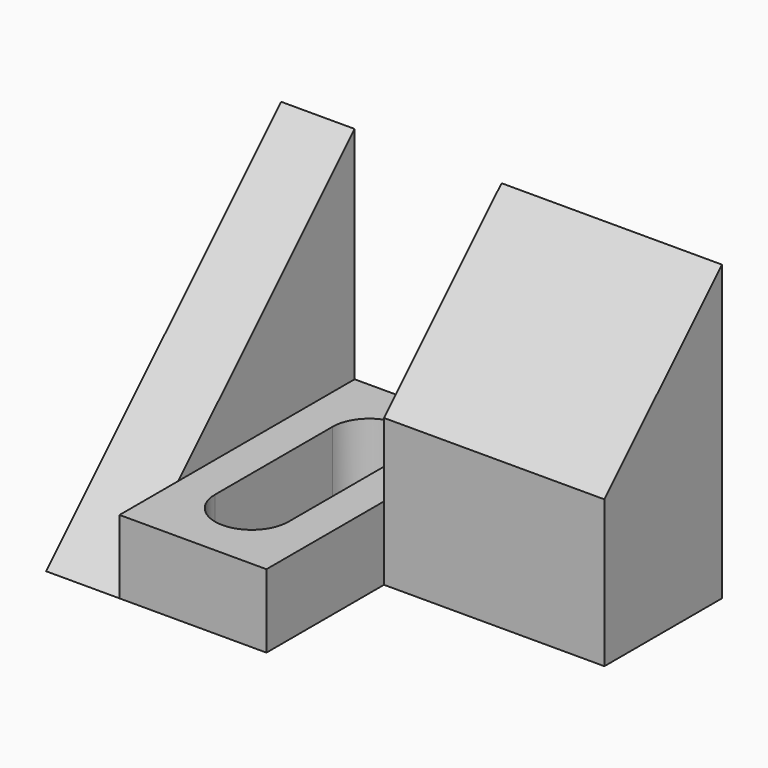
from build123d import *

# Parameters (mm, degrees)
F0_W     = 6.35
F0_H     = 25.4
F1_DEPTH = 25.4
F0_W_2   = 19.05
F0_H_2   = 12.7
F2_DEPTH = 25.4
F3_DEPTH = 6.35
F5_DEPTH = 38.101


# Not quite as in the source:
# - a feature of the source that left no trace in its solid (it failed there, or was rolled back) is left out


with BuildPart() as f1:
    # F0 (on Top) → F1 (new body)
    with BuildSketch(Plane.XY):
        with Locations((3.175, 12.7)):
            Rectangle(F0_W, F0_H)
    extrude(amount=F1_DEPTH)


with BuildPart() as f2:
    # F0 (on Top) → F2 (new body)
    with BuildSketch(Plane.XY):
        with Locations((28.575, 19.05)):
            Rectangle(F0_W_2, F0_H_2)
    extrude(amount=F2_DEPTH)


with BuildPart() as f3:
    # F0 (on Top) → F3 (new body)
    with BuildSketch(Plane.XY):
        Polygon((6.35, 25.4), (6.35, 0), (19.05, 0), (19.05, 12.7), (19.05, 25.4), align=None)
        with BuildLine():
            Line((9.525, 6.35), (9.525, 19.05))
            ThreePointArc((9.525, 19.05), (12.7, 22.225), (15.875, 19.05))
            Line((15.875, 19.05), (15.875, 6.35))
            ThreePointArc((15.875, 6.35), (12.7, 3.175), (9.525, 6.35))
        make_face(mode=Mode.SUBTRACT)
    extrude(amount=F3_DEPTH)


with BuildPart() as f5_tool:
    # F4 (on face) → F5 (new body, through all)
    with BuildSketch(Plane(origin=(0, 0, 0), x_dir=(0, -1, 0), z_dir=(-1, 0, 0))):
        Polygon((0, 25.4), (-25.4, 25.4), (0, 0), align=None)
    extrude(amount=-F5_DEPTH)


with BuildPart() as f1_1:
    add(f1.part)

    # F5: cut by f5_tool
    add(f5_tool.part, mode=Mode.SUBTRACT)


with BuildPart() as f2_1:
    add(f2.part)

    # F5: cut by f5_tool
    add(f5_tool.part, mode=Mode.SUBTRACT)


solid = Compound([f3.part, f1_1.part, f2_1.part])
